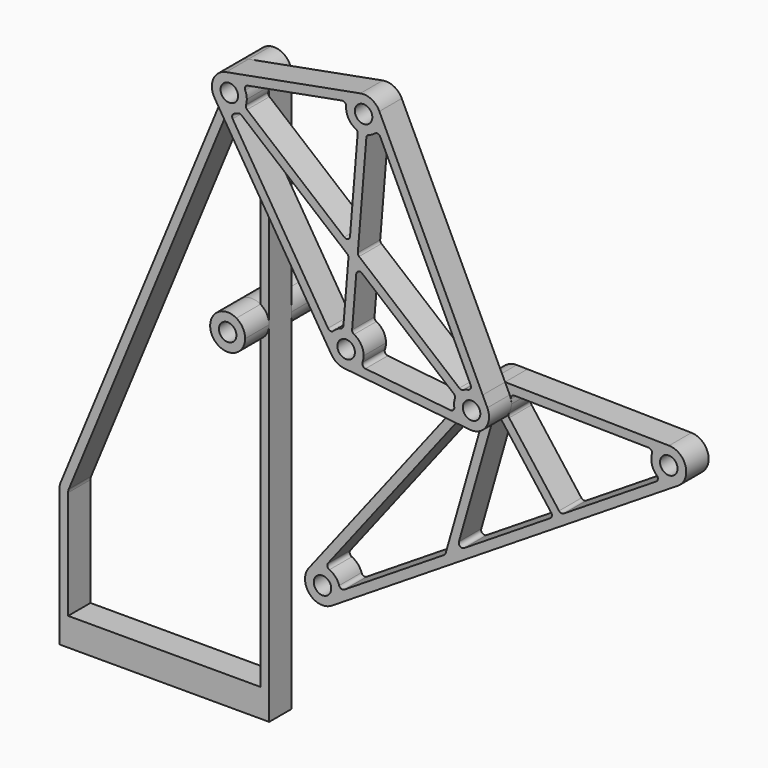
from build123d import *
from build123d import SkipClean  # not in build123d's __all__

# Parameters (mm, degrees)
F0_R      = 2.5
F1_DEPTH  = 8
F2_DEPTH  = 8
F3_DEPTH  = 8
F5_DEPTH  = 8.001
F7_DEPTH  = 16.001
F8_R      = 1
F9_R      = 1
F11_DEPTH = 8.001
F12_R     = 2.5
F13_DEPTH = 8.6
F14_R     = 2.5
F15_DEPTH = 8.6


# Not quite as in the source:
# - after a boolean that leaves OpenCascade's solid faulty, fix() repairs it
# - a feature names something its author has since deleted; it is built from what else it names


with BuildPart() as f1:
    # F0 (on Front) → F1 (new body)
    with BuildSketch(Plane.XZ):
        with BuildLine():
            Line((-60, 0), (0, 0))
            Line((0, 0), (0, 142.4990626805))
            Line((0, 142.4990626805), (-9.2453577588, 157.3586106875))
            ThreePointArc((-9.2453577588, 157.3586106875), (-9.9830566964, 159.5887264162), (-9.6209719225, 161.9096121311))
            Line((-9.6209719225, 161.9096121311), (-59.6209719225, 40.9171904993))
            ThreePointArc((-59.6209719225, 40.9171904993), (-59.904327661, 39.9810105402), (-60, 39.0075783681))
            Line((-60, 39.0075783681), (-60, 0))
        make_face()
        with Locations((-5, 100)):
            Circle(F0_R, mode=Mode.SUBTRACT)
        with BuildLine():
            Line((-9.2453577588, 157.3586106875), (0, 142.4990626805))
            Line((0, 142.4990626805), (0, 160))
            ThreePointArc((0, 160), (-1.8034272743, 163.8447266235), (-5.9127691238, 164.9159793049))
            ThreePointArc((-5.9127691238, 164.9159793049), (-8.1488304794, 163.8839241254), (-9.6209719225, 161.9096121311))
            ThreePointArc((-9.6209719225, 161.9096121311), (-9.9830566964, 159.5887264162), (-9.2453577588, 157.3586106875))
        make_face()
        with Locations((-5, 160)):
            Circle(F0_R, mode=Mode.SUBTRACT)
    extrude(amount=-F1_DEPTH)

    # F10 (on face) → F11 (cut, through all)
    with BuildSketch(Plane.XZ):
        with BuildLine():
            Line((-2.5, 104.3301270189), (-2.5, 155.6698729811))
            ThreePointArc((-2.5, 155.6698729811), (-5.9734321721, 155.095672339), (-8.9642585782, 156.9529269905))
            Line((-8.9642585782, 156.9529269905), (-57.3104859613, 39.9623844337))
            ThreePointArc((-57.3104859613, 39.9623844337), (-57.4521638305, 39.4942944542), (-57.5, 39.0075783681))
            Line((-57.5, 39.0075783681), (-57.5, 8))
            Line((-57.5, 8), (-2.5, 8))
            Line((-2.5, 8), (-2.5, 95.6698729811))
            ThreePointArc((-2.5, 95.6698729811), (-10, 100), (-2.5, 104.3301270189))
        make_face()
    extrude(amount=-F11_DEPTH, mode=Mode.SUBTRACT)

    # F12 (on face) → F13 (join)
    with BuildSketch(Plane.XZ):
        with BuildLine():
            ThreePointArc((-2.5, 95.6698729811), (-0.6698729811, 97.5), (0, 100))
            ThreePointArc((0, 100), (-0.6698729811, 102.5), (-2.5, 104.3301270189))
            ThreePointArc((-2.5, 104.3301270189), (-10, 100), (-2.5, 95.6698729811))
        make_face()
        with Locations((-5, 100)):
            Circle(F12_R, mode=Mode.SUBTRACT)
    with SkipClean():  # cleaning this boolean's faces spoils the solid; the shape is the same uncleaned
        extrude(amount=F13_DEPTH)

    # F14 (on face) → F15 (join)
    with BuildSketch(Plane(origin=(0, 8, 0), x_dir=(-1, 0, 0), z_dir=(0, 1, 0))):
        with BuildLine():
            ThreePointArc((2.5, 95.6698729811), (7.5, 95.6698729811), (10, 100))
            ThreePointArc((10, 100), (7.5, 104.3301270189), (2.5, 104.3301270189))
            ThreePointArc((2.5, 104.3301270189), (0.6698729811, 102.5), (0, 100))
            ThreePointArc((0, 100), (0.6698729811, 97.5), (2.5, 95.6698729811))
        make_face()
        with Locations((5, 100)):
            Circle(F14_R, mode=Mode.SUBTRACT)
    extrude(amount=F15_DEPTH)

    add(f1.part.fix(), mode=Mode.REPLACE)


with BuildPart() as f2:
    # F0 (on Front) → F2 (new body)
    with BuildSketch(Plane.XZ):
        with BuildLine():
            Line((0, 160), (0, 142.4990626805))
            Line((0, 142.4990626805), (24.1658678997, 103.6586106875))
            ThreePointArc((24.1658678997, 103.6586106875), (25.7580542129, 102.0619956016), (27.8898146222, 101.3272612645))
            Line((27.8898146222, 101.3272612645), (54.8134523133, 98.5042129253))
            Line((54.8134523133, 98.5042129253), (60.3189248798, 105.6040005326))
            ThreePointArc((60.3189248798, 105.6040005326), (62.1063069471, 107.0475744987), (64.3505759725, 107.5394047454))
            Line((64.3505759725, 107.5394047454), (67.4460449652, 107.489609955))
            Line((67.4460449652, 107.489609955), (37.9061104502, 169.2853672922))
            ThreePointArc((37.9061104502, 169.2853672922), (35.662352589, 171.5853242525), (32.4822566493, 172.0449340585))
            Line((32.4822566493, 172.0449340585), (-5.9127691238, 164.9159793049))
            ThreePointArc((-5.9127691238, 164.9159793049), (-1.8034272743, 163.8447266235), (0, 160))
        make_face()
        with Locations((28.4112256585, 106.3)):
            Circle(F0_R, mode=Mode.SUBTRACT)
        with Locations((33.3950257732, 167.1289547536)):
            Circle(F0_R, mode=Mode.SUBTRACT)
        with BuildLine():
            Line((60.3189248798, 105.6040005326), (54.8134523133, 98.5042129253))
            Line((54.8134523133, 98.5042129253), (63.7487436026, 97.5673128108))
            ThreePointArc((63.7487436026, 97.5673128108), (68.3549524812, 99.6565768043), (68.781239316, 104.6964640849))
            Line((68.781239316, 104.6964640849), (67.4460449652, 107.489609955))
            Line((67.4460449652, 107.489609955), (64.3505759725, 107.5394047454))
            ThreePointArc((64.3505759725, 107.5394047454), (62.1063069471, 107.0475744987), (60.3189248798, 105.6040005326))
        make_face()
        with Locations((64.2701546389, 102.5400515463)):
            Circle(F0_R, mode=Mode.SUBTRACT)
        with BuildLine():
            Line((-9.2453577588, 157.3586106875), (0, 142.4990626805))
            Line((0, 142.4990626805), (0, 160))
            ThreePointArc((0, 160), (-1.8034272743, 163.8447266235), (-5.9127691238, 164.9159793049))
            ThreePointArc((-5.9127691238, 164.9159793049), (-8.1488304794, 163.8839241254), (-9.6209719225, 161.9096121311))
            ThreePointArc((-9.6209719225, 161.9096121311), (-9.9830566964, 159.5887264162), (-9.2453577588, 157.3586106875))
        make_face()
        with Locations((-5, 160)):
            Circle(F0_R, mode=Mode.SUBTRACT)
    extrude(amount=F2_DEPTH)

    # F6 (on face) → F7 (cut, through all)
    with BuildSketch(Plane.XZ.offset(8)):
        with BuildLine():
            ThreePointArc((-2.0719137937, 155.9470614156), (-3.3830643017, 155.2686662612), (-4.8351686335, 155.0027176765))
            Line((-4.8351686335, 155.0027176765), (24.0010365332, 108.655893011))
            ThreePointArc((24.0010365332, 108.655893011), (25.4835070167, 110.3532041097), (27.560724067, 111.2271337553))
            Line((27.560724067, 111.2271337553), (29.1057757083, 130.085008111))
            Line((29.1057757083, 130.085008111), (-2.0719137937, 155.9470614156))
        make_face()
        with BuildLine():
            Line((28.6812782487, 168.796463157), (-1.1990215994, 163.2484709015))
            ThreePointArc((-1.1990215994, 163.2484709015), (-0.3093235028, 161.7313445637), (0, 160))
            ThreePointArc((0, 160), (-0.1204006605, 158.9093532716), (-0.4758041145, 157.8712323778))
            Line((-0.4758041145, 157.8712323778), (29.354965714, 133.1264558487))
            Line((29.354965714, 133.1264558487), (31.7538762933, 162.4059654052))
            ThreePointArc((31.7538762933, 162.4059654052), (28.8888306639, 164.962343197), (28.6812782487, 168.796463157))
        make_face()
        with BuildLine():
            ThreePointArc((37.5180761511, 164.3004470939), (36.0941205604, 162.9200490372), (34.2455273646, 162.2018209983))
            Line((34.2455273646, 162.2018209983), (31.7037157004, 131.1781556918))
            Line((31.7037157004, 131.1781556918), (61.3420684326, 106.5929901307))
            ThreePointArc((61.3420684326, 106.5929901307), (62.9173378165, 107.3535623903), (64.658188938, 107.5249717445))
            Line((64.658188938, 107.5249717445), (37.5180761511, 164.3004470939))
        make_face()
        with BuildLine():
            Line((31.4545256947, 128.1367079542), (30.0523751383, 111.0229893484))
            ThreePointArc((30.0523751383, 111.0229893484), (32.4858880616, 109.1977795465), (33.4112256585, 106.3))
            ThreePointArc((33.4112256585, 106.3), (33.1666994921, 104.7555037659), (32.4570382116, 103.362075429))
            Line((32.4570382116, 103.362075429), (59.7029310495, 100.5052373818))
            ThreePointArc((59.7029310495, 100.5052373818), (59.2704216119, 102.5917202881), (59.7459587534, 104.6688191685))
            Line((59.7459587534, 104.6688191685), (31.4545256947, 128.1367079542))
        make_face()
    extrude(amount=-F7_DEPTH, mode=Mode.SUBTRACT)

    # F8
    f8_edges = [f2.edges().sort_by_distance(p)[0] for p in [
        (-2.071914, -4, 155.947061),
        (-4.835169, -4, 155.002718),
        (-0.475804, -4, 157.871232),
        (-1.199022, -4, 163.248471),
        (28.681278, -4, 168.796463),
        (31.753876, -4, 162.405965),
        (34.245527, -4, 162.201821),
        (37.518076, -4, 164.300447),
        (29.354966, -4, 133.126456),
        (29.105776, -4, 130.085008),
        (31.454526, -4, 128.136708),
        (31.703716, -4, 131.178156),
        (27.560724, -4, 111.227134),
        (24.001037, -4, 108.655893),
        (30.052375, -4, 111.022989),
        (32.457038, -4, 103.362075),
        (59.702931, -4, 100.505237),
        (59.745959, -4, 104.668819),
        (61.342068, -4, 106.59299),
        (64.658189, -4, 107.524972),
    ]]
    fillet(f8_edges, radius=F8_R)


with BuildPart() as f3:
    # F0 (on Front) → F3 (new body)
    with BuildSketch(Plane.XZ):
        with BuildLine():
            Line((63.7487436026, 97.5673128108), (54.8134523133, 98.5042129253))
            Line((54.8134523133, 98.5042129253), (11.2957410983, 42.3843243873))
            ThreePointArc((11.2957410983, 42.3843243873), (11.5439415516, 35.9606769085), (17.913227288, 35.0905909328))
            Line((17.913227288, 35.0905909328), (116.9299430602, 97.506053742))
            ThreePointArc((116.9299430602, 97.506053742), (119.0782795725, 103.0847988452), (114.3441079633, 106.7351914092))
            Line((114.3441079633, 106.7351914092), (67.4460449652, 107.489609955))
            Line((67.4460449652, 107.489609955), (68.781239316, 104.6964640849))
            ThreePointArc((68.781239316, 104.6964640849), (68.3549524812, 99.6565768043), (63.7487436026, 97.5673128108))
        make_face()
        with Locations((15.2469708574, 39.3203754009)):
            Circle(F0_R, mode=Mode.SUBTRACT)
        with Locations((114.2636866297, 101.7358382101)):
            Circle(F0_R, mode=Mode.SUBTRACT)
        with BuildLine():
            Line((60.3189248798, 105.6040005326), (54.8134523133, 98.5042129253))
            Line((54.8134523133, 98.5042129253), (63.7487436026, 97.5673128108))
            ThreePointArc((63.7487436026, 97.5673128108), (68.3549524812, 99.6565768043), (68.781239316, 104.6964640849))
            Line((68.781239316, 104.6964640849), (67.4460449652, 107.489609955))
            Line((67.4460449652, 107.489609955), (64.3505759725, 107.5394047454))
            ThreePointArc((64.3505759725, 107.5394047454), (62.1063069471, 107.0475744987), (60.3189248798, 105.6040005326))
        make_face()
        with Locations((64.2701546389, 102.5400515463)):
            Circle(F0_R, mode=Mode.SUBTRACT)
    extrude(amount=-F3_DEPTH)

    # F4 (on face) → F5 (cut, through all)
    with BuildSketch(Plane.XZ):
        with BuildLine():
            Line((59.6410821013, 100.6501606919), (15.924813636, 44.2742152416))
            ThreePointArc((15.924813636, 44.2742152416), (18.9500001633, 42.6800738934), (20.2431998746, 39.5145289687))
            Line((20.2431998746, 39.5145289687), (50.3518725869, 58.4936147448))
            Line((50.3518725869, 58.4936147448), (61.7352488068, 98.2302658878))
            ThreePointArc((61.7352488068, 98.2302658878), (60.4893320781, 99.2681437292), (59.6410821013, 100.6501606919))
        make_face()
        with BuildLine():
            Line((64.1385780459, 97.5417830861), (53.5255211508, 60.4941329641))
            Line((53.5255211508, 60.4941329641), (81.3190963582, 78.0138905743))
            Line((81.3190963582, 78.0138905743), (66.2017264495, 97.9282156493))
            ThreePointArc((66.2017264495, 97.9282156493), (65.190658972, 97.6255147652), (64.1385780459, 97.5417830861))
        make_face()
        with BuildLine():
            Line((109.9743304236, 104.3051617275), (68.6399321786, 104.9700812279))
            ThreePointArc((68.6399321786, 104.9700812279), (69.1100352004, 103.7952631423), (69.2701546389, 102.5400515463))
            ThreePointArc((69.2701546389, 102.5400515463), (68.9931888298, 100.8990311224), (68.1929754262, 99.4398133183))
            Line((68.1929754262, 99.4398133183), (83.4419942953, 79.3520652068))
            Line((83.4419942953, 79.3520652068), (111.933714043, 97.3119001742))
            ThreePointArc((111.933714043, 97.3119001742), (109.4490936868, 100.386877575), (109.9743304236, 104.3051617275))
        make_face()
    extrude(amount=-F5_DEPTH, mode=Mode.SUBTRACT)

    # F9
    f9_edges = [f3.edges().sort_by_distance(p)[0] for p in [
        (15.924814, 4, 44.274215),
        (20.2432, 4, 39.514529),
        (111.933714, 4, 97.3119),
        (109.97433, 4, 104.305162),
        (68.192975, 4, 99.439813),
        (66.201726, 4, 97.928216),
        (64.138578, 4, 97.541783),
        (61.735249, 4, 98.230266),
        (59.641082, 4, 100.650161),
        (50.351873, 4, 58.493615),
        (53.525521, 4, 60.494133),
        (81.319096, 4, 78.013891),
        (68.639932, 4, 104.970081),
        (83.441994, 4, 79.352065),
    ]]
    fillet(f9_edges, radius=F9_R)


solid = Compound([f1.part, f2.part, f3.part])
